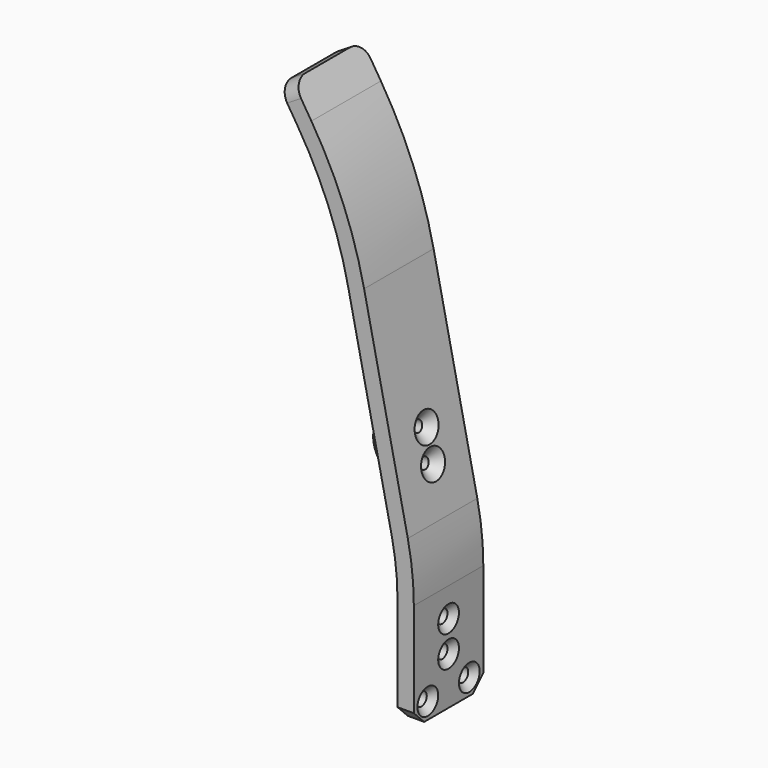
from build123d import *

# Parameters (mm, degrees)
F1_DEPTH        = 33.5
F2_R            = 6
F5_SIZE         = 5
F6_D            = 5.1
F6_CSINK_D      = 10
F6_CSINK_ANGLE  = 90
F7_W            = 8
F7_H            = 25
F8_DEPTH        = 12.5
F9_R            = 12.49999
F12_D           = 4.2
F12_DEPTH       = 13
F12_CSINK_D     = 11.2
F12_CSINK_ANGLE = 90
F12_TIP         = 1.2618073


# Not quite as in the source:
# - a fillet or chamfer is up to 0.001 mm smaller than in the source, because OpenCascade refuses the exact size


with BuildPart() as f1:
    # F0 (on Front) → F1 (new body)
    with BuildSketch(Plane.XZ):
        with BuildLine():
            Line((0, -25.4421804936), (0, -66.931756967))
            Line((0, -66.931756967), (6.3, -66.931756967))
            Line((6.3, -66.931756967), (6.3, -25.4421804936))
            ThreePointArc((6.3, -25.4421804936), (5.7176774776, -14.3308048482), (3.977089958, -3.3411677597))
            Line((3.977089958, -3.3411677597), (-12.8721835275, 75.928431603))
            ThreePointArc((-12.8721835275, 75.928431603), (-20.8378170534, 101.9828448791), (-33.2067360929, 126.2582153279))
            Line((-33.2067360929, 126.2582153279), (-40.38764708, 137.7500751305))
            Line((-40.38764708, 137.7500751305), (-45.7303500858, 134.4115837658))
            Line((-45.7303500858, 134.4115837658), (-38.5494390987, 122.9197239632))
            ThreePointArc((-38.5494390987, 122.9197239632), (-26.6790753372, 99.6228233406), (-19.0345134121, 74.6185879509))
            Line((-19.0345134121, 74.6185879509), (-2.1852399266, -4.6510114118))
            ThreePointArc((-2.1852399266, -4.6510114118), (-0.5478104632, -14.9893341668), (0, -25.4421804936))
        make_face()
    extrude(amount=F1_DEPTH)

    # F2
    f2_edges = [f1.edges().sort_by_distance(p)[0] for p in [
        (-43.058999, -33.5, 136.080829),
        (-43.058999, 0, 136.080829),
    ]]
    fillet(f2_edges, radius=F2_R)

    # F5
    f5_edges = [f1.edges().sort_by_distance(p)[0] for p in [
        (3.15, -33.5, -66.931757),
        (3.15, 0, -66.931757),
    ]]
    chamfer(f5_edges, length=F5_SIZE)

    # F6 (through all)
    with Locations(Plane.YZ.offset(6.3)):
        with Locations((-16.75, -36.631756967), (-16.75, -48.631756967), (-26.75, -60.631756967), (-6.75, -60.631756967)):
            CounterSinkHole(F6_D / 2, F6_CSINK_D / 2, counter_sink_angle=F6_CSINK_ANGLE)

    # F7 (on face) → F8 (join)
    with BuildSketch(Plane(origin=(-3.036646352, 0, -0.6454591076), x_dir=(0, -1, 0), z_dir=(-0.9781476007, 0, -0.2079116908))):
        with Locations((16.75, 19.5)):
            Rectangle(F7_W, F7_H)
    extrude(amount=F8_DEPTH)

    # F9 (radius 12.5 in the source; OpenCascade refuses exactly that, so slightly less here)
    f9_edges = [f1.edges().sort_by_distance(p)[0] for p in [
        (-16.718873, -16.75, 3.602678),
        (-21.916665, -16.75, 28.056368),
    ]]
    fillet(f9_edges, radius=F9_R)

    # F12
    with Locations(Plane(origin=(3.1256835326, 0, 0.6643845446), x_dir=(0, -1, 0), z_dir=(0.9781476007, 0, 0.2079116908))):
        with Locations((16.75, -25.5), (16.75, -13.5)):
            CounterSinkHole(F12_D / 2, F12_CSINK_D / 2, depth=F12_DEPTH, counter_sink_angle=F12_CSINK_ANGLE)
            with Locations((0, 0, -(F12_DEPTH + F12_TIP / 2))):  # 118° drill point
                Cone(0, F12_D / 2, F12_TIP, mode=Mode.SUBTRACT)


solid = f1.part
